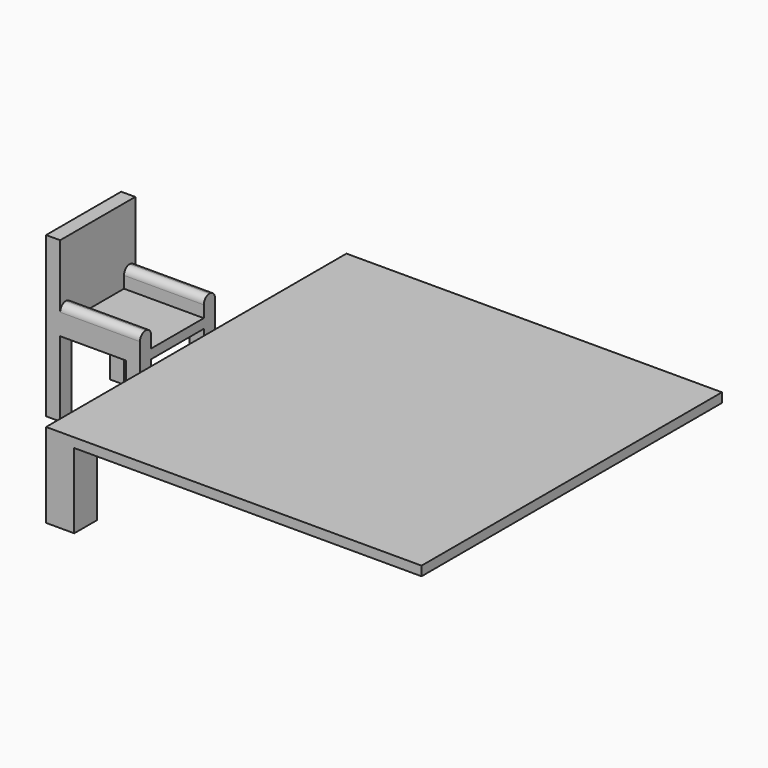
from build123d import *

# Parameters (mm, degrees)
F0_W      = 127
F0_H      = 127
F1_DEPTH  = 12.7
F2_W      = 19.05
F2_H      = 19.05
F3_DEPTH  = 101.6
F4_W      = 19.05
F4_H      = 127
F5_DEPTH  = 101.6
F6_W      = 107.95
F6_H      = 19.05
F7_DEPTH  = 25.4
F8_R      = 9.52499
F9_W      = 508
F9_H      = 508
F10_DEPTH = 12.7
F11_W     = 38.1
F11_H     = 38.1
F12_DEPTH = 101.6


# Not quite as in the source:
# - a fillet or chamfer is up to 0.001 mm smaller than in the source, because OpenCascade refuses the exact size


with BuildPart() as f1:
    # F0 (on Top) → F1 (new body)
    with BuildSketch(Plane.XY):
        with Locations((63.5, 63.5)):
            Rectangle(F0_W, F0_H)
    extrude(amount=F1_DEPTH)

    # F2 (on face) → F3 (join)
    with BuildSketch(Plane(origin=(0, 0, 0), x_dir=(1, 0, 0), z_dir=(0, 0, -1))):
        with Locations((9.525, -9.525)):
            Rectangle(F2_W, F2_H)
        with Locations((9.525, -117.475)):
            Rectangle(F2_W, F2_H)
        with Locations((117.475, -117.475)):
            Rectangle(F2_W, F2_H)
        with Locations((117.475, -9.525)):
            Rectangle(F2_W, F2_H)
    extrude(amount=F3_DEPTH)

    # F4 (on face) → F5 (join)
    with BuildSketch(Plane.XY.offset(12.7)):
        with Locations((9.525, 63.5)):
            Rectangle(F4_W, F4_H)
    extrude(amount=F5_DEPTH)

    # F6 (on face) → F7 (join)
    with BuildSketch(Plane.XY.offset(12.7)):
        with Locations((73.025, 9.525)):
            Rectangle(F6_W, F6_H)
        with Locations((73.025, 117.475)):
            Rectangle(F6_W, F6_H)
    extrude(amount=F7_DEPTH)

    # F8 (radius 9.525 in the source; OpenCascade refuses exactly that, so slightly less here)
    f8_edges = [f1.edges().sort_by_distance(p)[0] for p in [
        (73.025, 0, 38.1),
        (73.025, 19.05, 38.1),
        (73.025, 127, 38.1),
        (73.025, 107.95, 38.1),
    ]]
    fillet(f8_edges, radius=F8_R)


with BuildPart() as f10:
    # F9 (on Top) → F10 (new body)
    with BuildSketch(Plane.XY):
        with Locations((406.4, 63.5)):
            Rectangle(F9_W, F9_H)
    extrude(amount=F10_DEPTH)

    # F11 (on face) → F12 (join, through all)
    with BuildSketch(Plane(origin=(0, 0, 0), x_dir=(1, 0, 0), z_dir=(0, 0, -1))):
        with Locations((171.45, 171.45)):
            Rectangle(F11_W, F11_H)
    extrude(amount=F12_DEPTH)


solid = Compound([f1.part, f10.part])
